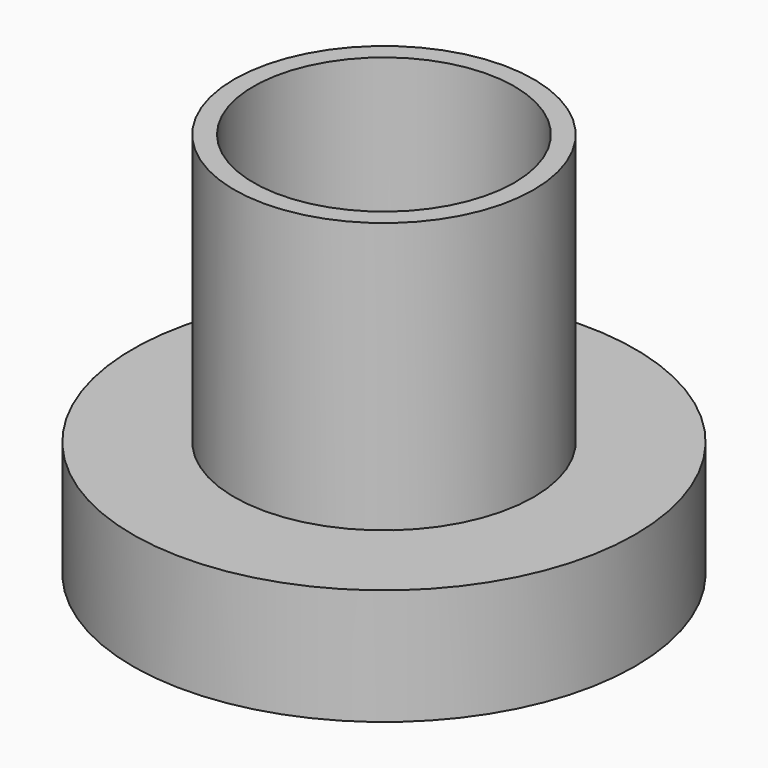
from build123d import *

# Parameters (mm, degrees)
F0_R     = 6.5
F0_R_2   = 3.875
F1_DEPTH = 3
F0_R_3   = 3.375
F2_DEPTH = 10


# Not quite as in the source:
# - a feature names something its author has since deleted; it is built from what else it names


with BuildPart() as f1:
    # F0 (on Top) → F1 (new body)
    with BuildSketch(Plane.XY):
        with Locations((-9.4900550321, 0)):
            Circle(F0_R)
        with Locations((-9.4900550321, 0)):
            Circle(F0_R_2, mode=Mode.SUBTRACT)
    extrude(amount=F1_DEPTH)


with BuildPart() as f2:
    # F0 (on Top) → F2 (new body)
    with BuildSketch(Plane.XY):
        with Locations((-9.4900550321, 0)):
            Circle(F0_R_2)
        with Locations((-9.4900550321, 0)):
            Circle(F0_R_3, mode=Mode.SUBTRACT)
    extrude(amount=F2_DEPTH)


solid = Compound([f1.part, f2.part])
